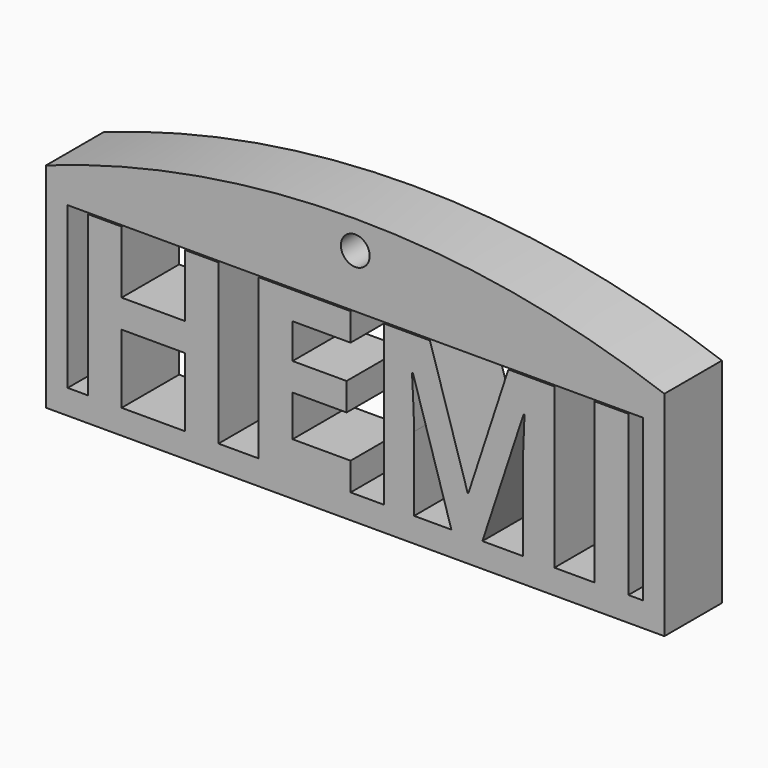
from build123d import *

# Parameters (mm, degrees)
F0_W         = 109.22
F0_H         = 37.7015848644
F0_R         = 2.54
F0_TEXT_SIZE = 39.4706810732
F1_DEPTH     = 12.7


# Not quite as in the source:
# - Text() gives the source's letters only with a copy of the font that has no kerning and outlines rounded to 1/6400 em; it was checked with that copy


with BuildPart() as f1:
    # F0 (on Front) → F1 (new body)
    with BuildSketch(Plane.XZ):
        with Locations((25.3587728447, 14.5172735211)):
            Rectangle(F0_W, F0_H)
        Polygon((-25.4343471273, 0), (-25.4343471273, 28.4188903727), (76.1656528727, 28.4188903727), (76.1656528727, 0), (73.6062258968, 0), (67.6301180906, 0), (60.5377300853, 0), (54.9686636776, 0), (47.820770027, 0), (42.3442130281, 0), (35.757543124, 0), (30.4166665913, 0), (24.5392354877, 0), (8.3130851903, 0), (1.2021953032, 0), (-4.7554106213, 0), (-15.9120453184, 0), (-21.8881531246, 0), align=None, mode=Mode.SUBTRACT)
        with BuildLine():
            ThreePointArc((79.9687728447, 33.3680659533), (25.3587728447, 42.8277307638), (-29.2512271553, 33.3680659533))
            Line((-29.2512271553, 33.3680659533), (79.9687728447, 33.3680659533))
        make_face()
        with Locations((25.3656528727, 37.8573313355)):
            Circle(F0_R, mode=Mode.SUBTRACT)
        with Locations((-25.4343471273, 0)):
            Text('HEMI', F0_TEXT_SIZE, font='Open Sans', font_style=FontStyle.BOLD, text_align=(TextAlign.LEFT, TextAlign.BOTTOM))
    extrude(amount=F1_DEPTH)


solid = f1.part
